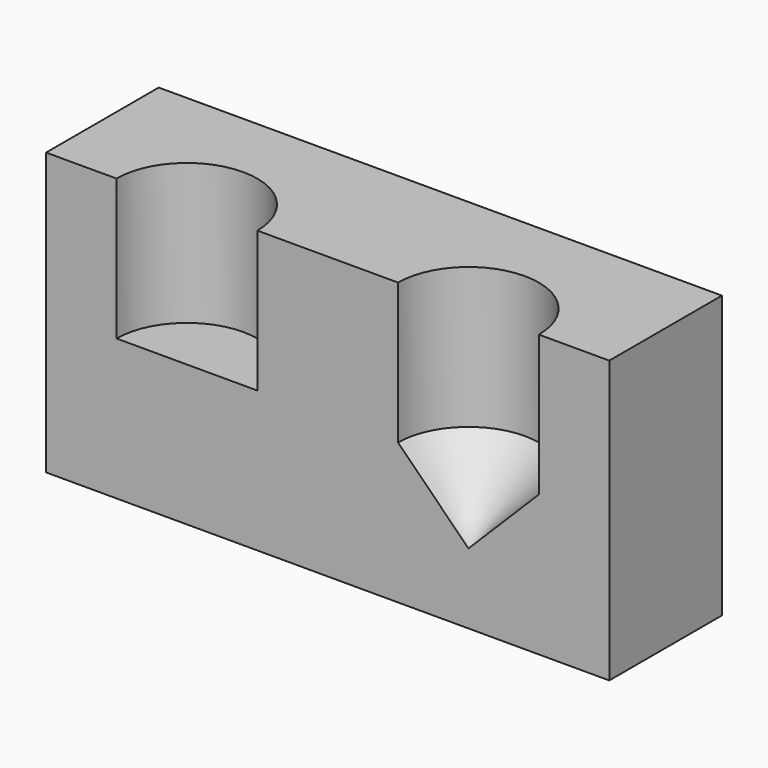
from build123d import *

# Parameters (mm, degrees)
F0_W     = 101.6
F0_H     = 50.8
F1_DEPTH = 50.8
F2_R     = 12.7
F3_DEPTH = 25.4
F5_R     = 12.7
F4_W     = 101.6
F4_H     = 25.4
F7_DEPTH = 50.8


# Not quite as in the source:
# - an extrude whose draft closes it to a point is written as a loft to that point


with BuildPart() as f1:
    # F0 (on Top) → F1 (new body)
    with BuildSketch(Plane.XY):
        Rectangle(F0_W, F0_H)
    extrude(amount=F1_DEPTH)

    # F2 (on face) → F3 (cut)
    with BuildSketch(Plane.XY.offset(50.8)):
        with Locations((-25.4, 0)):
            Circle(F2_R)
        with Locations((25.4, 0)):
            Circle(F2_R)
    extrude(amount=-F3_DEPTH, mode=Mode.SUBTRACT)

    # F5 (on face) → F6 section 0
    with BuildSketch(Plane.XY.offset(25.4), mode=Mode.PRIVATE) as f6_s0:
        with Locations((25.4, 0)):
            Circle(F5_R)
    loft([f6_s0.sketch, Vertex(25.4, 0, 12.7)], ruled=True, mode=Mode.SUBTRACT)

    # F4 (on face) → F7 (cut, through all)
    with BuildSketch(Plane.XY.offset(50.8)):
        with Locations((0, -12.7)):
            Rectangle(F4_W, F4_H)
    extrude(amount=-F7_DEPTH, mode=Mode.SUBTRACT)


solid = f1.part
